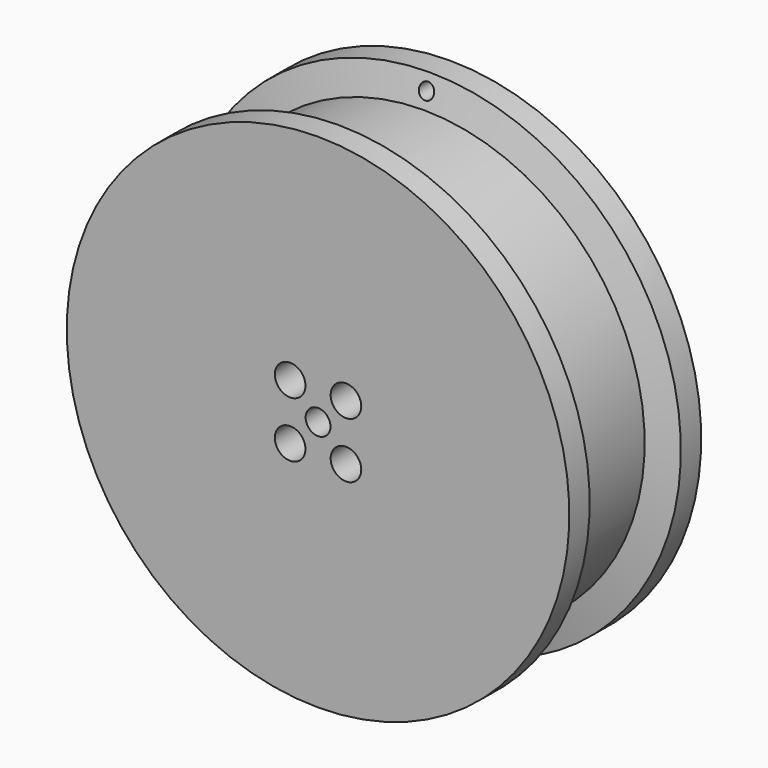
from build123d import *

# Parameters (mm, degrees)
F2_R         = 2.7768192656
F2_R_2       = 1.312388582
F3_DEPTH     = 28.9871403947
F4_SIZE      = 2
F5_R         = 3.418520713
F6_DEPTH     = 11.2
F7_S5_R      = 3.418520713
F7_T6_DEPTH  = 11
F7_S11_R     = 3.418520713
F7_T12_DEPTH = 11
F7_S17_R     = 3.418520713
F7_T18_DEPTH = 11
F7_S23_R     = 3.418520713
F7_T24_DEPTH = 11
F8_R         = 1.6764373153
F9_DEPTH     = 6.9756953811


# Not quite as in the source:
# - a fillet or chamfer that OpenCascade refuses, or shapes differently, is made with other operations: its cross-section is extruded or revolved along the edge and cut away or added


with BuildPart() as f1:
    # F0 (on Right) → F1 (revolve)
    with BuildSketch(Plane.YZ):
        Polygon((-18.4091031551, 56.1191700399), (-18.4091031551, 0), (10.5780372396, 0), (10.5780372396, 17.1244889498), (18.4091031551, 17.1244889498), (18.4091031551, 56.1191700399), (12.7344317734, 56.1191700399), (11.0015068203, 49.418527633), (0, 49.418527633), (-11.0015068203, 49.418527633), (-12.7344317734, 56.1191700399), align=None)
    revolve(axis=Axis((0, 11.9474316016, 0), (0, 1, 0)))

    # F2 (on face) → F3 (cut, through all)
    with BuildSketch(Plane(origin=(0, 10.5780372396, 0), x_dir=(-1, 0, 0), z_dir=(0, 1, 0))):
        Circle(F2_R)
        with Locations((-6.2308004126, 6.2308004126)):
            Circle(F2_R_2)
        with Locations((6.2308004126, 6.2308004126)):
            Circle(F2_R_2)
        with Locations((6.2308004126, -6.2308004126)):
            Circle(F2_R_2)
        with Locations((-6.2308004126, -6.2308004126)):
            Circle(F2_R_2)
    extrude(amount=-F3_DEPTH, mode=Mode.SUBTRACT)

    # F4
    f4_edges = [f1.edges().sort_by_distance(p)[0] for p in [
        (0, 18.409103, -17.124489),
    ]]
    chamfer(f4_edges, length=F4_SIZE)

    # F5 (on face) → F6 (cut)
    with BuildSketch(Plane.XZ.offset(18.4091031551)):
        with Locations((-6.2308004126, 6.2308004126)):
            Circle(F5_R)
        with Locations((6.2308004126, 6.2308004126)):
            Circle(F5_R)
        with Locations((6.2308004126, -6.2308004126)):
            Circle(F5_R)
        with Locations((-6.2308004126, -6.2308004126)):
            Circle(F5_R)
    extrude(amount=-F6_DEPTH, mode=Mode.SUBTRACT)

    # F7: chamfer of 5 on 4 edges, made by hand


with BuildPart() as f7_tool2:
    # F7_s3 → F7_t4 (revolve)
    with BuildSketch(Plane.XY.offset(6.2308004126)):
        Polygon((-7.5431889946, -2.2091031551), (-12.5431889946, -7.2091031551), (-7.5431889946, -7.2091031551), align=None)
    revolve(axis=Axis((-6.2308004126, -7.2091031551, 6.2308004126), (0, 1, 0)))

    # F7_s5 → F7_t6 (intersect, symmetric)
    with BuildSketch(Plane.XZ.offset(4.7)):
        with Locations((-6.2308004126, 6.2308004126)):
            Circle(F7_S5_R)
    extrude(amount=F7_T6_DEPTH, both=True, mode=Mode.INTERSECT)


with BuildPart() as f1_1:
    add(f1.part)

    # F7_t1: cut F7_tool2
    add(f7_tool2.part, mode=Mode.SUBTRACT)


with BuildPart() as f7_tool8:
    # F7_s9 → F7_t10 (revolve)
    with BuildSketch(Plane.XY.offset(-6.2308004126)):
        Polygon((-7.5431889946, -2.2091031551), (-12.5431889946, -7.2091031551), (-7.5431889946, -7.2091031551), align=None)
    revolve(axis=Axis((-6.2308004126, -7.2091031551, -6.2308004126), (0, 1, 0)))

    # F7_s11 → F7_t12 (intersect, symmetric)
    with BuildSketch(Plane.XZ.offset(4.7)):
        with Locations((-6.2308004126, -6.2308004126)):
            Circle(F7_S11_R)
    extrude(amount=F7_T12_DEPTH, both=True, mode=Mode.INTERSECT)


with BuildPart() as f1_2:
    add(f1_1.part)

    # F7_t7: cut F7_tool8
    add(f7_tool8.part, mode=Mode.SUBTRACT)


with BuildPart() as f7_tool14:
    # F7_s15 → F7_t16 (revolve)
    with BuildSketch(Plane.XY.offset(-6.2308004126)):
        Polygon((4.9184118305, -2.2091031551), (-0.0815881695, -7.2091031551), (4.9184118305, -7.2091031551), align=None)
    revolve(axis=Axis((6.2308004126, -7.2091031551, -6.2308004126), (0, 1, 0)))

    # F7_s17 → F7_t18 (intersect, symmetric)
    with BuildSketch(Plane.XZ.offset(4.7)):
        with Locations((6.2308004126, -6.2308004126)):
            Circle(F7_S17_R)
    extrude(amount=F7_T18_DEPTH, both=True, mode=Mode.INTERSECT)


with BuildPart() as f1_3:
    add(f1_2.part)

    # F7_t13: cut F7_tool14
    add(f7_tool14.part, mode=Mode.SUBTRACT)


with BuildPart() as f7_tool20:
    # F7_s21 → F7_t22 (revolve)
    with BuildSketch(Plane.XY.offset(6.2308004126)):
        Polygon((4.9184118305, -2.2091031551), (-0.0815881695, -7.2091031551), (4.9184118305, -7.2091031551), align=None)
    revolve(axis=Axis((6.2308004126, -7.2091031551, 6.2308004126), (0, 1, 0)))

    # F7_s23 → F7_t24 (intersect, symmetric)
    with BuildSketch(Plane.XZ.offset(4.7)):
        with Locations((6.2308004126, 6.2308004126)):
            Circle(F7_S23_R)
    extrude(amount=F7_T24_DEPTH, both=True, mode=Mode.INTERSECT)


with BuildPart() as f1_4:
    add(f1_3.part)

    # F7_t19: cut F7_tool20
    add(f7_tool20.part, mode=Mode.SUBTRACT)

    # F8 (on face) → F9 (cut, through all)
    with BuildSketch(Plane(origin=(0, 18.4091031551, 0), x_dir=(-1, 0, 0), z_dir=(0, 1, 0))):
        with Locations((0, 52.7688488364)):
            Circle(F8_R)
    extrude(amount=-F9_DEPTH, mode=Mode.SUBTRACT)


solid = f1_4.part
